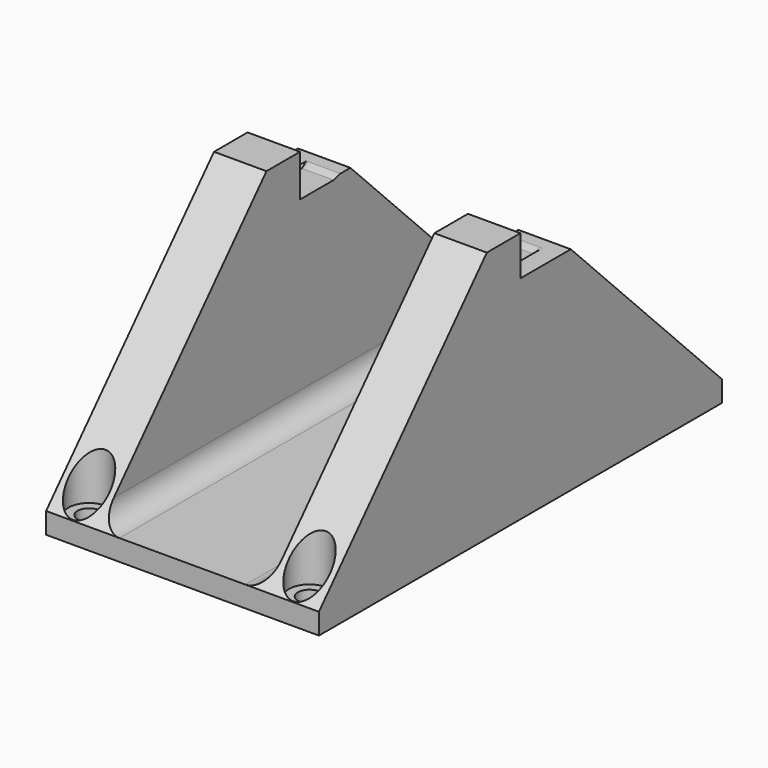
from build123d import *

# Parameters (mm, degrees)
F1_DEPTH       = 32.5
F2_W           = 40
F2_H           = 55
F3_DEPTH       = 60.001
F3_DEPTH_BACK  = 60.001
F4_R           = 5
F6_D           = 5.5
F6_START       = 44.8625
F6_START_2     = 44.8735114
F6_CBORE_D     = 9.75
F6_CBORE_DEPTH = 1
F7_W           = 5
F7_H           = 12
F8_DEPTH       = 0.5358983849
F9_T4_DEPTH    = 13.5430097928
F9_T10_DEPTH   = 13.5430097928


# Not quite as in the source:
# - a fillet or chamfer that OpenCascade refuses, or shapes differently, is made with other operations: its cross-section is extruded or revolved along the edge and cut away or added


with BuildPart() as f1:
    # F0 (on Right) → F1 (new body, symmetric)
    with BuildSketch(Plane.YZ):
        Polygon((0, 50), (0, 60), (-10, 60), (-60, 5), (-60, 0), (60, 0), (60, 5), (15, 50.5358983849), (12, 50.5358983849), (10, 50), align=None)
    extrude(amount=F1_DEPTH, both=True)

    # F2 (on Front) → F3 (cut, two sides)
    with BuildSketch(Plane.XZ) as f3_sk:
        with Locations((0, 32.5)):
            Rectangle(F2_W, F2_H)
    extrude(amount=-F3_DEPTH, mode=Mode.SUBTRACT)
    extrude(f3_sk.sketch, amount=F3_DEPTH_BACK, mode=Mode.SUBTRACT)

    # F4
    f4_edges = [f1.edges().sort_by_distance(p)[0] for p in [
        (20, 0, 5),
        (-20, 0, 5),
    ]]
    fillet(f4_edges, radius=F4_R)

    # F6 (through all)
    # its depths count from where the whole tool has entered the part; down to there all is cleared
    with Locations(Plane.XY.offset(50)):
        with Locations((-26.25, 55, -F6_START_2), (26.25, 55, -F6_START_2), (-26.25, -55, -F6_START), (26.25, -55, -F6_START)):
            CounterBoreHole(F6_D / 2, F6_CBORE_D / 2, F6_CBORE_DEPTH)

    # F7 (on face) → F8 (join, through all)
    with BuildSketch(Plane.XY.offset(50)):
        with Locations((-30, 6)):
            Rectangle(F7_W, F7_H)
        with Locations((30, 6)):
            Rectangle(F7_W, F7_H)
    extrude(amount=F8_DEPTH)

    # F9: chamfer of 0.6 on 2 edges, made by hand


with BuildPart() as f9_tool2:
    # F9_s3 → F9_t4 (new body)
    with BuildSketch(Plane.XZ.offset(-13.5430097928)):
        Polygon((27.5, 49.9358983849), (28.1, 50.5358983849), (27.5, 50.5358983849), align=None)
    extrude(amount=F9_T4_DEPTH)

    split(bisect_by=Plane(origin=(0, -11.8301270189, 44.1506350946), x_dir=(1, 0, 0), z_dir=(0, -0.2588190451, 0.9659258263)), keep=Keep.TOP)

    split(bisect_by=Plane.XY.offset(50), keep=Keep.TOP)


with BuildPart() as f1_1:
    add(f1.part)

    # F9_t1: cut F9_tool2
    add(f9_tool2.part, mode=Mode.SUBTRACT)


with BuildPart() as f9_tool8:
    # F9_s9 → F9_t10 (new body)
    with BuildSketch(Plane.XZ):
        Polygon((-27.5, 49.9358983849), (-28.1, 50.5358983849), (-27.5, 50.5358983849), align=None)
    extrude(amount=-F9_T10_DEPTH)

    split(bisect_by=Plane(origin=(0, -11.8301270189, 44.1506350946), x_dir=(1, 0, 0), z_dir=(0, -0.2588190451, 0.9659258263)), keep=Keep.TOP)

    split(bisect_by=Plane.XY.offset(50), keep=Keep.TOP)


with BuildPart() as f1_2:
    add(f1_1.part)

    # F9_t7: cut F9_tool8
    add(f9_tool8.part, mode=Mode.SUBTRACT)


solid = f1_2.part
